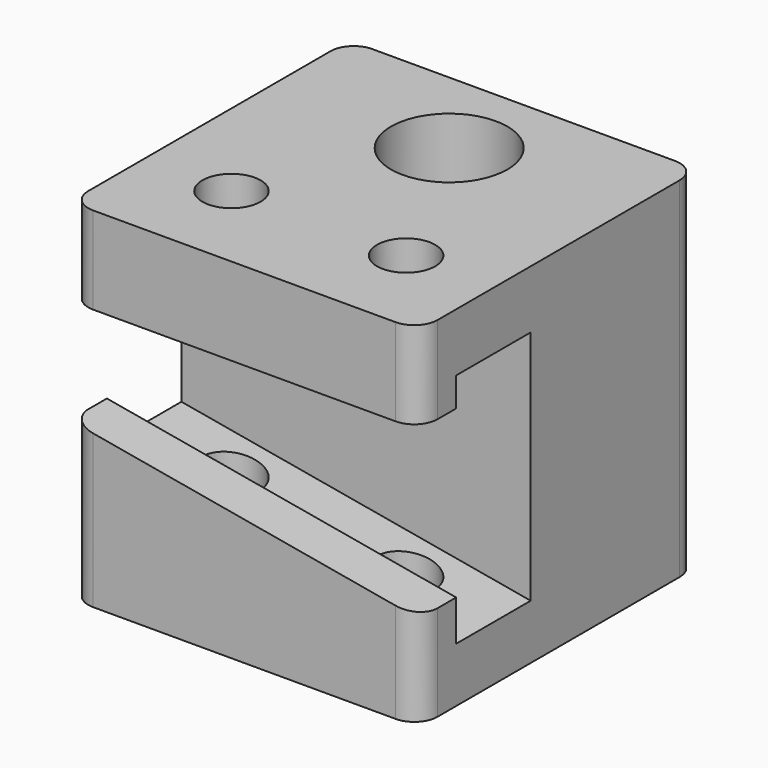
from build123d import *

# Parameters (mm, degrees)
F0_W     = 76.2
F0_H     = 76.2
F1_DEPTH = 76.2
F6_R     = 6.35
F6_R_2   = 12.7
F7_DEPTH = 76.2010001
F8_R     = 5.08


with BuildPart() as f1:
    # F0 (on Top) → F1 (new body)
    with BuildSketch(Plane.XY):
        Rectangle(F0_W, F0_H)
    extrude(amount=F1_DEPTH)

    # F2 (on face) → F5 section 0
    with BuildSketch(Plane(origin=(-38.1, 0, 0), x_dir=(0, -1, 0), z_dir=(-1, 0, 0))):
        Polygon((38.1, 34.29), (38.1, 57.15), (27.94, 57.15), (27.94, 63.5), (7.62, 63.5), (7.62, 25.4), (27.94, 25.4), (27.94, 34.29), align=None)
    # F4 (on face) → F5 section 1
    with BuildSketch(Plane.YZ.offset(38.1)):
        Polygon((-27.94, 57.15), (-38.1, 57.15), (-38.1, 20.85388407), (-27.94, 20.85388407), (-27.94, 11.96388407), (-7.62, 11.96388407), (-7.62, 63.5), (-27.94, 63.5), align=None)
    loft(mode=Mode.SUBTRACT)

    # F6 (on face) → F7 (cut, through all)
    with BuildSketch(Plane.XY.offset(76.2)):
        with Locations((-19.05, -17.78)):
            Circle(F6_R)
        with Locations((19.05, -17.78)):
            Circle(F6_R)
        with Locations((0, 17.78)):
            Circle(F6_R_2)
    extrude(amount=-F7_DEPTH, mode=Mode.SUBTRACT)

    # F8
    f8_edges = [f1.edges().sort_by_distance(p)[0] for p in [
        (38.1, 38.1, 38.1),
        (-38.1, 38.1, 38.1),
        (38.1, -38.1, 10.426942),
        (-38.1, -38.1, 17.145),
        (38.1, -38.1, 66.675),
        (-38.1, -38.1, 66.675),
    ]]
    fillet(f8_edges, radius=F8_R)


solid = f1.part
